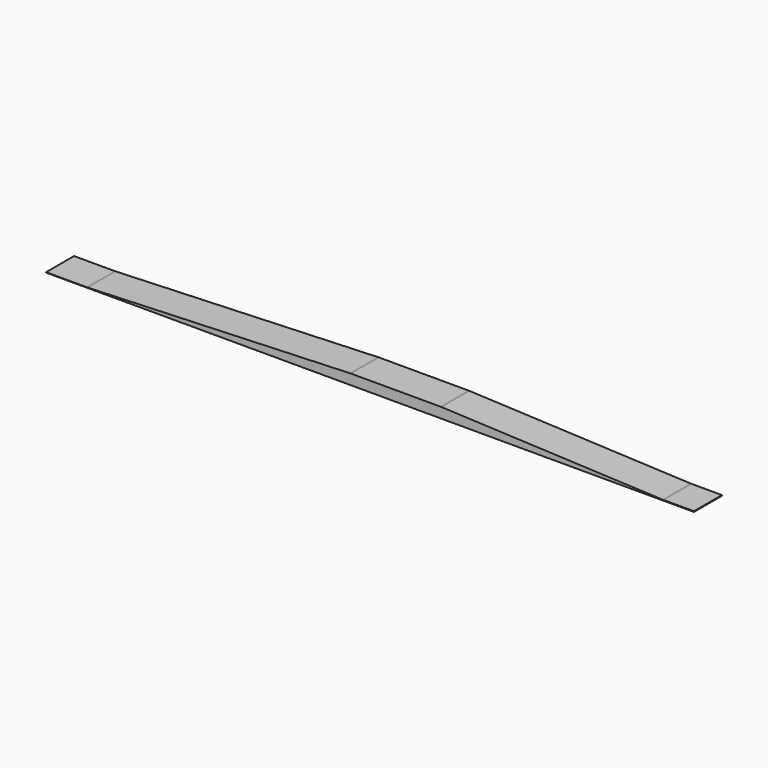
from build123d import *

# Parameters (mm, degrees)
F1_DEPTH    = 107.95
F2_T1_DEPTH = 107.95
F3_T1_DEPTH = 107.95
F3_T3_DEPTH = 115.0912402897
F3_T5_DEPTH = 116.2011283703


# Not quite as in the source:
# - a fillet or chamfer that OpenCascade refuses, or shapes differently, is made with other operations: its cross-section is extruded or revolved along the edge and cut away or added


with BuildPart() as f1:
    # F0 (on Front) → F1 (new body)
    with BuildSketch(Plane.XZ):
        Polygon((-1016, 1.27), (-1016, 0), (984, 0), (984, 2.032), (889, 2.032), (203.2, 31.75), (-76.2, 31.75), (-889, 1.27), align=None)
    extrude(amount=F1_DEPTH)

    # F2: fillet of radius 76.2 on 1 edges, made by hand

    # F2_s2 → F2_t1 (join)
    with BuildSketch(Plane.XZ):
        with BuildLine():
            ThreePointArc((-887.5727551211, 1.323521683), (-889.0002508168, 1.2833815957), (-890.4282480579, 1.27))
            Line((-890.4282480579, 1.27), (-889, 1.27))
            Line((-889, 1.27), (-887.5727551211, 1.323521683))
        make_face()
    extrude(amount=F2_T1_DEPTH)

    # F3: fillet of radius 76.2 on 3 edges, made by hand

    # F3_s2 → F3_t1 (join)
    with BuildSketch(Plane.XZ):
        with BuildLine():
            ThreePointArc((890.6502256741, 2.032), (889.0003868453, 2.0498627772), (887.3513215259, 2.1034427339))
            Line((887.3513215259, 2.1034427339), (889, 2.032))
            Line((889, 2.032), (890.6502256741, 2.032))
        make_face()
    extrude(amount=F3_T1_DEPTH)

    # F3_s4 → F3_t3 (cut)
    with BuildSketch(Plane.XZ.offset(-3.5706201449)):
        with BuildLine():
            ThreePointArc((-77.6272448789, 31.696478317), (-76.1997491832, 31.7366184043), (-74.7717519421, 31.75))
            Line((-74.7717519421, 31.75), (-76.2, 31.75))
            Line((-76.2, 31.75), (-77.6272448789, 31.696478317))
        make_face()
    extrude(amount=F3_T3_DEPTH, mode=Mode.SUBTRACT)

    # F3_s6 → F3_t5 (cut)
    with BuildSketch(Plane.XZ.offset(-4.1255641851)):
        with BuildLine():
            ThreePointArc((201.5497743259, 31.75), (203.1996131547, 31.7321372228), (204.8486784741, 31.6785572661))
            Line((204.8486784741, 31.6785572661), (203.2, 31.75))
            Line((203.2, 31.75), (201.5497743259, 31.75))
        make_face()
    extrude(amount=F3_T5_DEPTH, mode=Mode.SUBTRACT)


solid = f1.part
